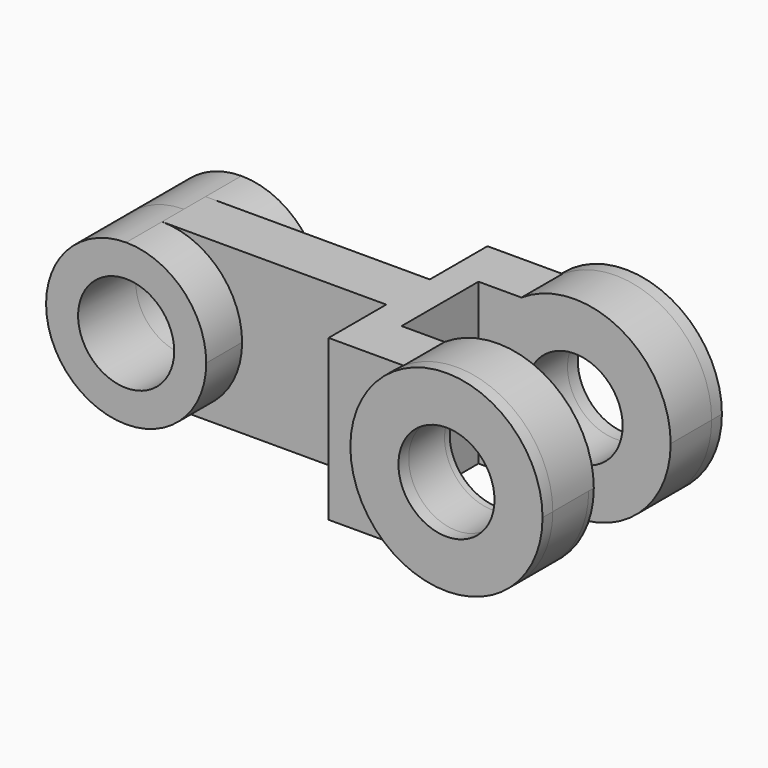
from build123d import *

# Parameters (mm, degrees)
F0_R      = 15
F1_DEPTH  = 22.5
F2_DEPTH  = 8.5
F5_W      = 10
F5_H      = 50
F6_DEPTH  = 31
F8_R      = 15
F9_DEPTH  = 16
F10_DEPTH = 14
F12_DEPTH = 4


# Not quite as in the source:
# - a pattern or mirror of a feature is missing from the dataset's text; its kind, count and spacing are read off the source's solid


with BuildPart() as f1:
    # F0 (on Front) → F1 (new body, symmetric)
    with BuildSketch(Plane.XZ):
        with BuildLine():
            ThreePointArc((0, -25), (17.6776695297, -17.6776695297), (25, 0))
            ThreePointArc((25, 0), (17.6776695297, 17.6776695297), (0, 25))
            ThreePointArc((0, 25), (-25, 0), (0, -25))
        make_face()
        Circle(F0_R, mode=Mode.SUBTRACT)
    extrude(amount=F1_DEPTH, both=True)

    # F0 (on Front) → F2 (join, symmetric)
    with BuildSketch(Plane.XZ):
        with BuildLine():
            ThreePointArc((0, 25), (17.6776695297, 17.6776695297), (25, 0))
            ThreePointArc((25, 0), (17.6776695297, -17.6776695297), (0, -25))
            Line((0, -25), (70, -25))
            Line((70, -25), (70, 25))
            Line((70, 25), (0, 25))
        make_face()
    extrude(amount=F2_DEPTH, both=True)

    # F5 (on Front) → F6 (join, symmetric)
    with BuildSketch(Plane.XZ):
        with Locations((75, 0)):
            Rectangle(F5_W, F5_H)
    extrude(amount=F6_DEPTH, both=True)

    # F8 (on face) → F9 (join)
    with BuildSketch(Plane.XZ.offset(31)):
        with BuildLine():
            Line((93.4168760482, 25), (80, 25))
            Line((80, 25), (80, 0))
            ThreePointArc((80, 0), (83.5661796315, 14.1863716546), (93.4168760482, 25))
        make_face()
        with BuildLine():
            ThreePointArc((93.4168760482, 25), (83.5661796315, 14.1863716546), (80, 0))
            ThreePointArc((80, 0), (83.5661796315, -14.1863716546), (93.4168760482, -25))
            ThreePointArc((93.4168760482, -25), (124.1863716546, -26.4338203685), (140, 0))
            ThreePointArc((140, 0), (124.1863716546, 26.4338203685), (93.4168760482, 25))
        make_face()
        with Locations((110, 0)):
            Circle(F8_R, mode=Mode.SUBTRACT)
        with BuildLine():
            ThreePointArc((93.4168760482, -25), (83.5661796315, -14.1863716546), (80, 0))
            Line((80, 0), (80, -25))
            Line((80, -25), (93.4168760482, -25))
        make_face()
    f9 = extrude(amount=-F9_DEPTH)

    # F9_copies: F9 across plane
    add(f9.mirror(Plane.ZX))

    # F8 (on face) → F10 (join)
    with BuildSketch(Plane.XZ.offset(31)):
        with BuildLine():
            Line((93.4168760482, 25), (80, 25))
            Line((80, 25), (80, 0))
            ThreePointArc((80, 0), (83.5661796315, 14.1863716546), (93.4168760482, 25))
        make_face()
        with BuildLine():
            ThreePointArc((93.4168760482, -25), (83.5661796315, -14.1863716546), (80, 0))
            Line((80, 0), (80, -25))
            Line((80, -25), (93.4168760482, -25))
        make_face()
        with BuildLine():
            ThreePointArc((93.4168760482, 25), (83.5661796315, 14.1863716546), (80, 0))
            ThreePointArc((80, 0), (83.5661796315, -14.1863716546), (93.4168760482, -25))
            ThreePointArc((93.4168760482, -25), (124.1863716546, -26.4338203685), (140, 0))
            ThreePointArc((140, 0), (124.1863716546, 26.4338203685), (93.4168760482, 25))
        make_face()
        with Locations((110, 0)):
            Circle(F8_R, mode=Mode.SUBTRACT)
    extrude(amount=-F10_DEPTH)

    # F8 (on face) → F12 (join)
    with BuildSketch(Plane.XZ.offset(31)):
        with BuildLine():
            ThreePointArc((93.4168760482, 25), (83.5661796315, 14.1863716546), (80, 0))
            ThreePointArc((80, 0), (83.5661796315, -14.1863716546), (93.4168760482, -25))
            ThreePointArc((93.4168760482, -25), (124.1863716546, -26.4338203685), (140, 0))
            ThreePointArc((140, 0), (124.1863716546, 26.4338203685), (93.4168760482, 25))
        make_face()
        with Locations((110, 0)):
            Circle(F8_R, mode=Mode.SUBTRACT)
    f12 = extrude(amount=F12_DEPTH)

    # F12_copies: F12 across plane
    add(f12.mirror(Plane.ZX))


solid = f1.part
